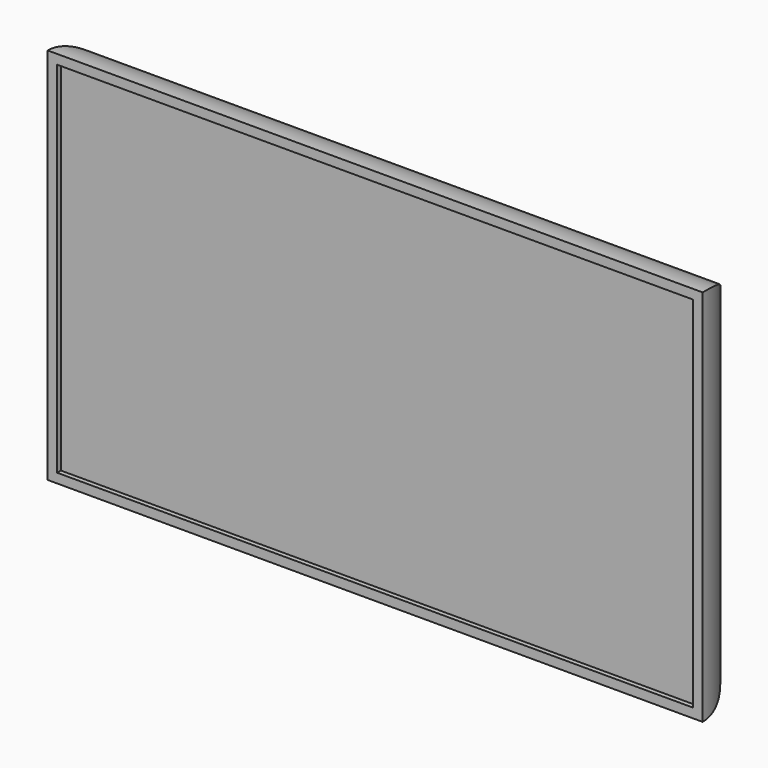
from build123d import *

# Parameters (mm, degrees)
F0_W     = 263.9645430735
F0_H     = 152.4
F1_DEPTH = 25.4
F2_W     = 256.3445430735
F2_H     = 144.78
F3_DEPTH = 1.905
F4_R     = 25.39999


# Not quite as in the source:
# - a fillet or chamfer is up to 0.001 mm smaller than in the source, because OpenCascade refuses the exact size


with BuildPart() as f1:
    # F0 (on Front) → F1 (new body)
    with BuildSketch(Plane.XZ):
        with Locations((-0.0032023633, -16.0101552037)):
            Rectangle(F0_W, F0_H)
    extrude(amount=F1_DEPTH)

    # F2 (on face) → F3 (cut)
    with BuildSketch(Plane.XZ.offset(25.4)):
        with Locations((-0.0032023633, -16.0101552037)):
            Rectangle(F2_W, F2_H)
    extrude(amount=-F3_DEPTH, mode=Mode.SUBTRACT)

    # F4 (radius 25.4 in the source; OpenCascade refuses exactly that, so slightly less here)
    f4_edges = [f1.edges().sort_by_distance(p)[0] for p in [
        (-0.003202, 0, -92.210155),
        (131.979069, 0, -16.010155),
        (-0.003202, 0, 60.189845),
        (-131.985474, 0, -16.010155),
    ]]
    fillet(f4_edges, radius=F4_R)


solid = f1.part
